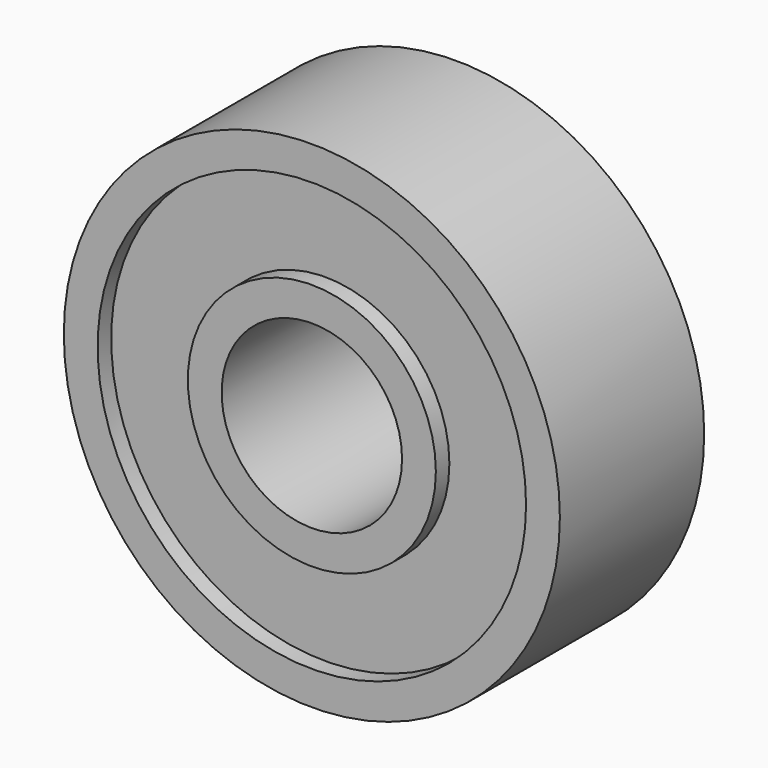
from build123d import *

# Parameters (mm, degrees)
F0_R     = 11
F0_R_2   = 9.5
F1_DEPTH = 4
F2_R     = 5.5
F2_R_2   = 4
F3_DEPTH = 4
F4_R     = 9.5
F4_R_2   = 5.5
F5_DEPTH = 3.25


with BuildPart() as f1:
    # F0 (on Front) → F1 (new body, symmetric)
    with BuildSketch(Plane.XZ):
        Circle(F0_R)
        Circle(F0_R_2, mode=Mode.SUBTRACT)
    extrude(amount=F1_DEPTH, both=True)



with BuildPart() as f3:
    # F2 (on Front) → F3 (new body, symmetric)
    with BuildSketch(Plane.XZ):
        Circle(F2_R)
        Circle(F2_R_2, mode=Mode.SUBTRACT)
    extrude(amount=F3_DEPTH, both=True)


with BuildPart() as f1_1:
    add(f1.part)

    add(f3.part)  # F5 merges F3
    # F4 (on Front) → F5 (join, symmetric)
    with BuildSketch(Plane.XZ):
        Circle(F4_R)
        Circle(F4_R_2, mode=Mode.SUBTRACT)
    extrude(amount=F5_DEPTH, both=True)


solid = f1_1.part
